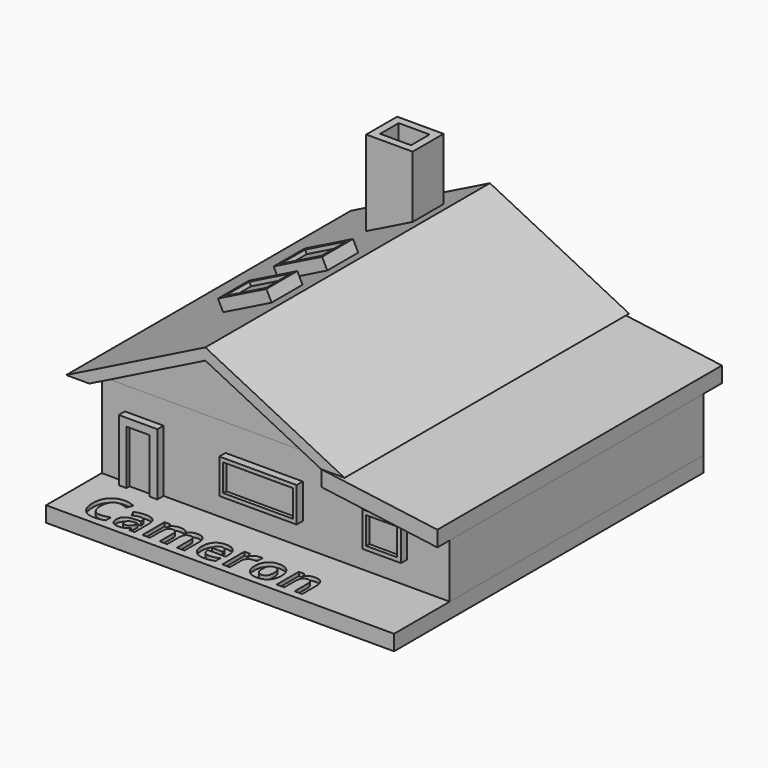
from build123d import *

# Parameters (mm, degrees)
F1_DEPTH       = 914.4
F1_DEPTH_BACK  = 13106.4
F2_DEPTH       = 304.8
F2_DEPTH_BACK  = 12192
F0_W           = 4572
F0_H           = 609.6
F3_DEPTH       = 3048
F3_DEPTH_BACK  = 12192
F0_W_2         = 3048
F0_H_2         = 1371.6
F0_W_3         = 1524
F0_W_4         = 2743.2
F0_H_3         = 1066.8
F0_W_5         = 1219.2
F0_W_6         = 914.4
F0_H_4         = 2133.6
F4_DEPTH       = 304.8
F4_DEPTH_BACK  = 12192
F5_DEPTH       = 457.2
F6_DEPTH       = 609.6
F7_W           = 1219.2
F7_H           = 1066.8
F8_DEPTH       = 457.2
F7_W_2         = 1524
F7_H_2         = 1371.6
F10_DEPTH      = 609.6
F11_DEPTH      = 609.6
F12_DEPTH      = 457.2
F13_W          = 1828.8
F13_H          = 1524
F13_W_2        = 1219.2
F13_H_2        = 914.4
F14_DEPTH      = 8839.2
F9_W           = 2133.6
F9_H           = 1524
F9_W_2         = 1828.8
F9_H_2         = 1219.2
F15_DEPTH      = 457.2
F16_DEPTH      = 304.8
F17_W          = 2743.2
F17_H          = 1524
F17_W_2        = 2438.4
F17_H_2        = 1219.2
F18_DEPTH      = 609.6
F18_DEPTH_BACK = 609.6
F19_DEPTH      = 457.2
F19_DEPTH_BACK = 457.2
F20_TEXT_SIZE  = 2000.1508692763
F21_DEPTH      = 152.4


# Not quite as in the source:
# - Text() gives the source's letters only with a copy of the font that has no kerning and outlines rounded to 1/6400 em; it was checked with that copy


with BuildPart() as f1:
    # F0 (on Front) → F1 (new body, two sides)
    with BuildSketch(Plane.XZ) as f1_sk:
        Polygon((-5486.4, 0), (-4572, 0), (0, 2286), (0, 2743.2), align=None)
        Polygon((0, 2286), (4572, 0), (5486.4, 0), (0, 2743.2), align=None)
    extrude(amount=F1_DEPTH)
    extrude(f1_sk.sketch, amount=-F1_DEPTH_BACK)



with BuildPart() as f1b:
    # F0 (on Front) → F1, piece 2 (new body, two sides)
    with BuildSketch(Plane.XZ) as f1_2_sk:
        Polygon((9144, -609.6), (4572, 0), (4572, -614.9947954251), (9144, -1224.5947954251), align=None)
    extrude(amount=F1_DEPTH)
    extrude(f1_2_sk.sketch, amount=-F1_DEPTH_BACK)


with BuildPart() as f1_1:
    add(f1.part)

    add(f1b.part)  # F2 merges F1b
    # F0 (on Front) → F2 (join, two sides)
    with BuildSketch(Plane.XZ) as f2_sk:
        Polygon((-4572, 0), (0, 0), (0, 2286), align=None)
        Polygon((0, 2286), (0, 0), (4572, 0), align=None)
    extrude(amount=F2_DEPTH)
    extrude(f2_sk.sketch, amount=-F2_DEPTH_BACK)

    # F9 (on face) → F15 (join)
    with BuildSketch(Plane(origin=(-1097.28, 0, 2194.56), x_dir=(0.894427191, 0, 0.4472135955), z_dir=(-0.4472135955, 0, 0.894427191))):
        with Locations((-602.0036648245, 6705.6)):
            Rectangle(F9_W, F9_H)
        with Locations((-602.0036648245, 6705.6)):
            Rectangle(F9_W_2, F9_H_2, mode=Mode.SUBTRACT)
        with Locations((-602.0036648245, 3962.4)):
            Rectangle(F9_W, F9_H)
        with Locations((-602.0036648245, 3962.4)):
            Rectangle(F9_W_2, F9_H_2, mode=Mode.SUBTRACT)
    extrude(amount=F15_DEPTH)

    # F16 (add): faces of the model
    f16_faces = [f1_1.faces().sort_by_distance(p)[0] for p in [
        (-1635.7284469006, 6705.6, 1925.3357765497),
        (-1635.7284469006, 3962.4, 1925.3357765497),
    ]]
    extrude(f16_faces, amount=F16_DEPTH)


with BuildPart() as f3:
    # F0 (on Front) → F3 (new body, two sides)
    with BuildSketch(Plane.XZ) as f3_sk:
        Polygon((-3657.6, -3352.8), (-4572, -3352.8), (-4572, -3962.4), (4572, -3962.4), (4572, -3352.8), (-2133.6, -3352.8), (-2438.4, -3352.8), (-3352.8, -3352.8), align=None)
        with Locations((6858, -3657.6)):
            Rectangle(F0_W, F0_H)
    extrude(amount=F3_DEPTH)
    extrude(f3_sk.sketch, amount=-F3_DEPTH_BACK)

    # F20 (on face) → F21 (cut)
    with BuildSketch(Plane.XY.offset(-3352.8)):
        with Locations((-3657.6, -2743.2)):
            Text('Cameron', F20_TEXT_SIZE, font='Open Sans', font_style=FontStyle.BOLD, text_align=(TextAlign.LEFT, TextAlign.BOTTOM))
    extrude(amount=-F21_DEPTH, mode=Mode.SUBTRACT)


with BuildPart() as f4:
    # F0 (on Front) → F4 (new body, two sides)
    with BuildSketch(Plane.XZ) as f4_sk:
        Polygon((4572, 0), (0, 0), (-4572, 0), (-4572, -3352.8), (-3657.6, -3352.8), (-3657.6, -914.4), (-2133.6, -914.4), (-2133.6, -3352.8), (4572, -3352.8), (4572, -614.9947954251), align=None)
        with Locations((1828.8, -1752.6)):
            Rectangle(F0_W_2, F0_H_2, mode=Mode.SUBTRACT)
        Polygon((9144, -1224.5947954251), (4572, -614.9947954251), (4572, -3352.8), (9144, -3352.8), align=None)
        with Locations((6705.6, -1752.6)):
            Rectangle(F0_W_3, F0_H_2, mode=Mode.SUBTRACT)
        with Locations((1828.8, -1752.6)):
            Rectangle(F0_W_2, F0_H_2)
        with Locations((1828.8, -1752.6)):
            Rectangle(F0_W_4, F0_H_3, mode=Mode.SUBTRACT)
        with Locations((1828.8, -1752.6)):
            Rectangle(F0_W_4, F0_H_3)
        with Locations((6705.6, -1752.6)):
            Rectangle(F0_W_3, F0_H_2)
        with Locations((6705.6, -1752.6)):
            Rectangle(F0_W_5, F0_H_3, mode=Mode.SUBTRACT)
        with Locations((-2895.6, -2286)):
            Rectangle(F0_W_6, F0_H_4)
        Polygon((-3657.6, -914.4), (-3657.6, -3352.8), (-3352.8, -3352.8), (-3352.8, -1219.2), (-2438.4, -1219.2), (-2438.4, -3352.8), (-2133.6, -3352.8), (-2133.6, -914.4), align=None)
        with Locations((6705.6, -1752.6)):
            Rectangle(F0_W_5, F0_H_3)
    extrude(amount=F4_DEPTH)
    extrude(f4_sk.sketch, amount=-F4_DEPTH_BACK)

    # F7 (on face) → F8 (join)
    with BuildSketch(Plane(origin=(-4572, 0, 0), x_dir=(0, -1, 0), z_dir=(-1, 0, 0))):
        with Locations((-9448.8, -1752.6)):
            Rectangle(F7_W, F7_H)
    extrude(amount=F8_DEPTH)

    # F7 (on face) → F10 (join)
    with BuildSketch(Plane(origin=(-4572, 0, 0), x_dir=(0, -1, 0), z_dir=(-1, 0, 0))):
        with Locations((-9448.8, -1752.6)):
            Rectangle(F7_W_2, F7_H_2)
        with Locations((-9448.8, -1752.6)):
            Rectangle(F7_W, F7_H, mode=Mode.SUBTRACT)
    extrude(amount=F10_DEPTH)

    # F7 (on face) → F11 (join)
    with BuildSketch(Plane(origin=(-4572, 0, 0), x_dir=(0, -1, 0), z_dir=(-1, 0, 0))):
        with Locations((-9448.8, -1752.6)):
            Rectangle(F7_W_2, F7_H_2)
        with Locations((-9448.8, -1752.6)):
            Rectangle(F7_W, F7_H, mode=Mode.SUBTRACT)
        with Locations((-2438.4, -1752.6)):
            Rectangle(F7_W_2, F7_H_2)
        with Locations((-2438.4, -1752.6)):
            Rectangle(F7_W, F7_H, mode=Mode.SUBTRACT)
    extrude(amount=F11_DEPTH)

    # F12 (add): a face of the model
    f12_faces = [f4.faces().sort_by_distance(p)[0] for p in [
        (-4572, 2438.4, -1752.6),
    ]]
    extrude(f12_faces, amount=F12_DEPTH)

    # F17 (on face) → F18 (join, two sides)
    with BuildSketch(Plane(origin=(0, 12192, 0), x_dir=(-1, 0, 0), z_dir=(0, 1, 0))) as f18_sk:
        with Locations((-3139.44, -1828.8)):
            Rectangle(F17_W, F17_H)
        with Locations((-3139.44, -1828.8)):
            Rectangle(F17_W_2, F17_H_2, mode=Mode.SUBTRACT)
    extrude(amount=F18_DEPTH)
    extrude(f18_sk.sketch, amount=-F18_DEPTH_BACK)

    # F19 (add, two sides): a face of the model
    f19_faces = [f4.faces().sort_by_distance(p)[0] for p in [
        (3139.44, 12192, -1828.8),
    ]]
    extrude(f19_faces, amount=F19_DEPTH)
    extrude(f19_faces, amount=-F19_DEPTH_BACK)


with BuildPart() as f5:
    # F0 (on Front) → F5 (new body)
    with BuildSketch(Plane.XZ):
        with Locations((-2895.6, -2286)):
            Rectangle(F0_W_6, F0_H_4)
    extrude(amount=F5_DEPTH)


with BuildPart() as f5b:
    # F0 (on Front) → F5, piece 2 (new body)
    with BuildSketch(Plane.XZ):
        with Locations((1828.8, -1752.6)):
            Rectangle(F0_W_4, F0_H_3)
    extrude(amount=F5_DEPTH)


with BuildPart() as f5c:
    # F0 (on Front) → F5, piece 3 (new body)
    with BuildSketch(Plane.XZ):
        with Locations((6705.6, -1752.6)):
            Rectangle(F0_W_5, F0_H_3)
    extrude(amount=F5_DEPTH)


with BuildPart() as f6:
    # F0 (on Front) → F6 (new body)
    with BuildSketch(Plane.XZ):
        Polygon((-3657.6, -914.4), (-3657.6, -3352.8), (-3352.8, -3352.8), (-3352.8, -1219.2), (-2438.4, -1219.2), (-2438.4, -3352.8), (-2133.6, -3352.8), (-2133.6, -914.4), align=None)
    extrude(amount=F6_DEPTH)


with BuildPart() as f6b:
    # F0 (on Front) → F6, piece 2 (new body)
    with BuildSketch(Plane.XZ):
        with Locations((1828.8, -1752.6)):
            Rectangle(F0_W_2, F0_H_2)
        with Locations((1828.8, -1752.6)):
            Rectangle(F0_W_4, F0_H_3, mode=Mode.SUBTRACT)
    extrude(amount=F6_DEPTH)


with BuildPart() as f6c:
    # F0 (on Front) → F6, piece 3 (new body)
    with BuildSketch(Plane.XZ):
        with Locations((6705.6, -1752.6)):
            Rectangle(F0_W_3, F0_H_2)
        with Locations((6705.6, -1752.6)):
            Rectangle(F0_W_5, F0_H_3, mode=Mode.SUBTRACT)
    extrude(amount=F6_DEPTH)


with BuildPart() as f14:
    # F13 (on face) → F14 (new body)
    with BuildSketch(Plane(origin=(0, 0, -3962.4), x_dir=(1, 0, 0), z_dir=(0, 0, -1))):
        with Locations((-1524, -10820.4)):
            Rectangle(F13_W, F13_H)
        with Locations((-1524, -10820.4)):
            Rectangle(F13_W_2, F13_H_2, mode=Mode.SUBTRACT)
    extrude(amount=-F14_DEPTH)


solid = Compound([f1_1.part, f3.part, f4.part, f5.part, f5b.part, f5c.part, f6.part, f6b.part, f6c.part, f14.part])
